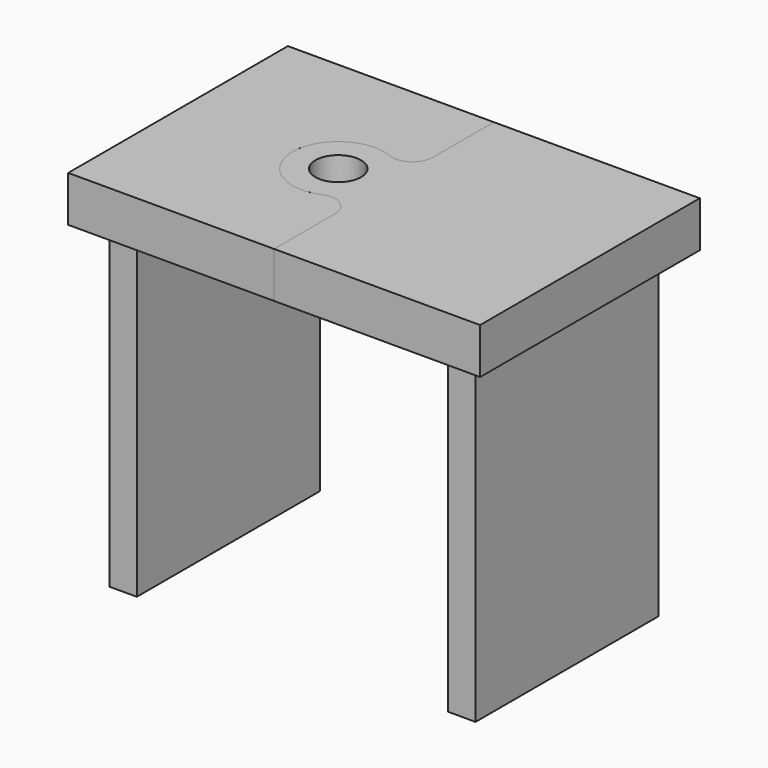
from build123d import *

# Parameters (mm, degrees)
F1_DEPTH = 10
F2_R     = 5
F3_DEPTH = 10
F4_W     = 6
F4_H     = 50
F5_DEPTH = 70


with BuildPart() as f1:
    # F0 (on Top) → F1 (new body)
    with BuildSketch(Plane.XY):
        with BuildLine():
            Line((0, 60), (0, 0))
            Line((0, 0), (45, 0))
            Line((45, 0), (45, 16.625795157))
            ThreePointArc((45, 16.625795157), (43.2056172384, 20.2215753726), (39.2534953958, 20.9497084623))
            ThreePointArc((39.2534953958, 20.9497084623), (25, 30), (39.2534953958, 39.0502915377))
            ThreePointArc((39.2534953958, 39.0502915377), (43.2056172384, 39.7784246274), (45, 43.374204843))
            Line((45, 43.374204843), (45, 60))
            Line((45, 60), (0, 60))
        make_face()
    extrude(amount=F1_DEPTH)

    # F4 (on Top) → F5 (join)
    with BuildSketch(Plane.XY):
        with Locations((8, 30)):
            Rectangle(F4_W, F4_H)
    extrude(amount=-F5_DEPTH)


with BuildPart() as f3:
    # F2 (on Top) → F3 (new body)
    with BuildSketch(Plane.XY):
        with BuildLine():
            ThreePointArc((38.3439909876, 39.4243155866), (38.788495333, 39.2123841147), (39.2534953958, 39.0502915377))
            ThreePointArc((39.2534953958, 39.0502915377), (38.8033437044, 39.2484905074), (38.3439909876, 39.4243155866))
        make_face()
        with BuildLine():
            ThreePointArc((45, 43.374204843), (43.2056172384, 39.7784246274), (39.2534953958, 39.0502915377))
            ThreePointArc((39.2534953958, 39.0502915377), (38.788495333, 39.2123841147), (38.3439909876, 39.4243155866))
            ThreePointArc((38.3439909876, 39.4243155866), (25, 30), (38.3439909876, 20.5756844134))
            ThreePointArc((38.3439909876, 20.5756844134), (38.788495333, 20.7876158853), (39.2534953958, 20.9497084623))
            ThreePointArc((39.2534953958, 20.9497084623), (43.2056172384, 20.2215753726), (45, 16.625795157))
            Line((45, 16.625795157), (45, 0))
            Line((45, 0), (90, 0))
            Line((90, 0), (90, 60))
            Line((90, 60), (45, 60))
            Line((45, 60), (45, 43.374204843))
        make_face()
        with Locations((35, 30)):
            Circle(F2_R, mode=Mode.SUBTRACT)
        with BuildLine():
            ThreePointArc((39.2534953958, 20.9497084623), (38.788495333, 20.7876158853), (38.3439909876, 20.5756844134))
            ThreePointArc((38.3439909876, 20.5756844134), (38.8033437044, 20.7515094926), (39.2534953958, 20.9497084623))
        make_face()
    extrude(amount=F3_DEPTH)

    # F4 (on Top) → F5, piece 2 (join)
    with BuildSketch(Plane.XY):
        with Locations((82, 30)):
            Rectangle(F4_W, F4_H)
    extrude(amount=-F5_DEPTH)


solid = Compound([f1.part, f3.part])
